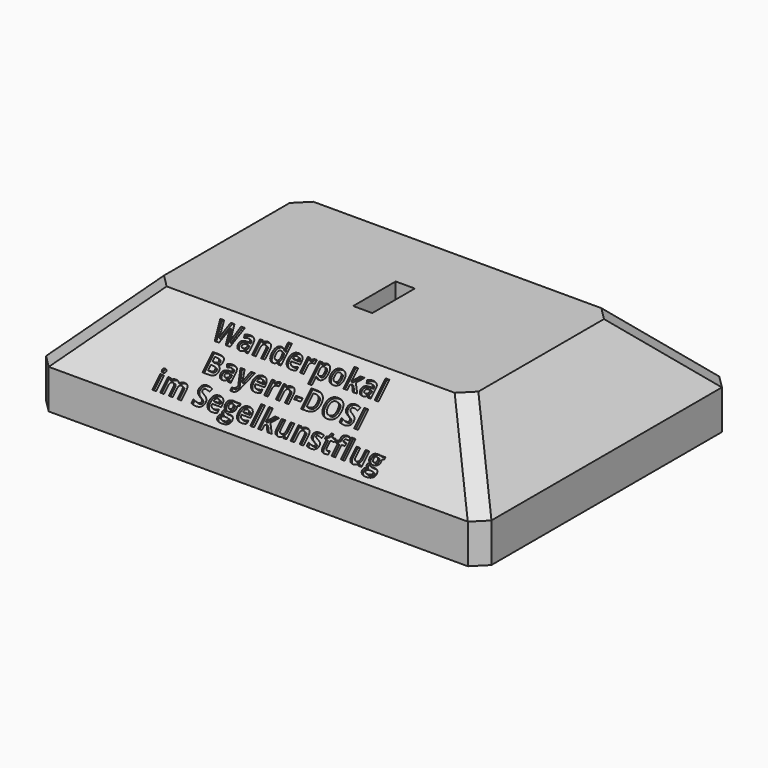
from build123d import *

# Parameters (mm, degrees)
F0_W         = 170
F0_H         = 120
F1_DEPTH     = 40
F2_SIZE      = 25
F3_SIZE      = 5
F6_TEXT_SIZE = 9.7222222222
F7_DEPTH     = 1
F8_W         = 7.3
F8_H         = 20.3
F9_DEPTH     = 20
F10_SIZE     = 4.1


# Not quite as in the source:
# - Text() gives the source's letters only with a copy of the font that has no kerning and outlines rounded to 1/6400 em; it was checked with that copy


with BuildPart() as f1:
    # F0 (on Top) → F1 (new body)
    with BuildSketch(Plane.XY):
        Rectangle(F0_W, F0_H)
    extrude(amount=F1_DEPTH)

    # F2
    f2_edges = [f1.edges().sort_by_distance(p)[0] for p in [
        (0, 60, 40),
        (-85, 0, 40),
        (0, -60, 40),
        (85, 0, 40),
    ]]
    chamfer(f2_edges, length=F2_SIZE)

    # F3
    f3_edges = [f1.edges().sort_by_distance(p)[0] for p in [
        (-85, -60, 7.5),
        (-85, 60, 7.5),
        (85, -60, 7.5),
        (85, 60, 7.5),
    ]]
    chamfer(f3_edges, length=F3_SIZE)

    # F6 (on offset) → F7 (cut)
    with BuildSketch(Plane(origin=(0, -37.5, 37.5), x_dir=(1, 0, 0), z_dir=(0, -0.7071067812, 0.7071067812))):
        with Locations((-32.4425998264, -7)):
            Text('Wanderpokal', F6_TEXT_SIZE, font='Open Sans', font_style=FontStyle.BOLD, text_align=(TextAlign.LEFT, TextAlign.BOTTOM))
        with Locations((-30.4389105903, -17.2222222222)):
            Text('Bayern-DOSI', F6_TEXT_SIZE, font='Open Sans', font_style=FontStyle.BOLD, text_align=(TextAlign.LEFT, TextAlign.BOTTOM))
        with Locations((-43.6656901042, -27.4444444444)):
            Text('im Segelkunstflug', F6_TEXT_SIZE, font='Open Sans', font_style=FontStyle.BOLD, text_align=(TextAlign.LEFT, TextAlign.BOTTOM))
    extrude(amount=-F7_DEPTH, mode=Mode.SUBTRACT)

    # F8 (on face) → F9 (cut)
    with BuildSketch(Plane.XY.offset(40)):
        Rectangle(F8_W, F8_H)
    extrude(amount=-F9_DEPTH, mode=Mode.SUBTRACT)

    # F10
    f10_edges = [f1.edges().sort_by_distance(p)[0] for p in [
        (-71.25, -46.25, 28.75),
        (71.25, -46.25, 28.75),
        (-71.25, 46.25, 28.75),
        (71.25, 46.25, 28.75),
    ]]
    chamfer(f10_edges, length=F10_SIZE)


solid = f1.part
